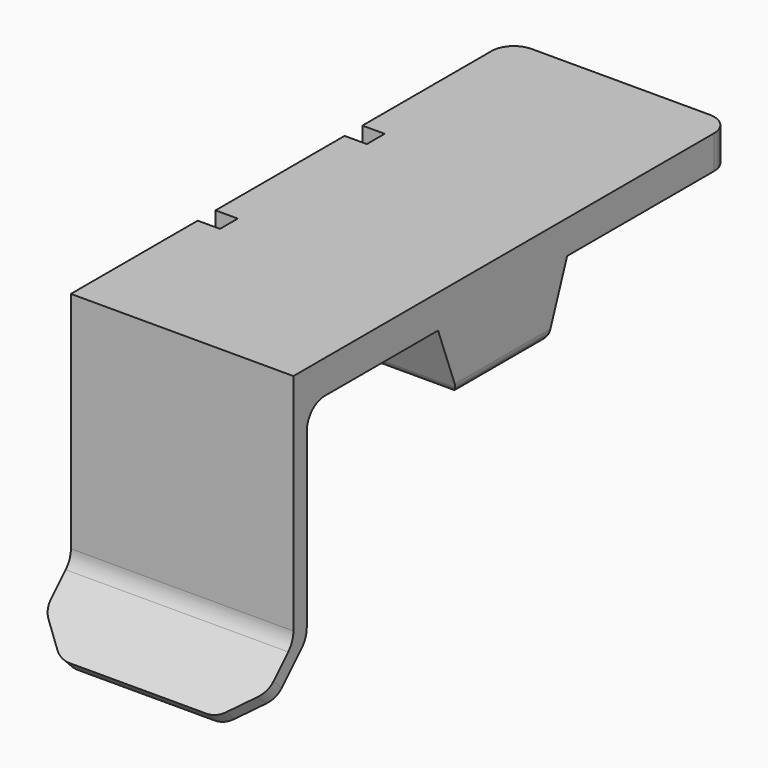
from build123d import *

# Parameters (mm, degrees)
F0_W         = 20
F0_H         = 47.7648153901
F1_DEPTH     = 3
F3_W         = 20
F3_H         = 23
F4_DEPTH     = 1.5
F5_T1_DEPTH  = 30.2867319519
F6_W         = 20
F6_H         = 2.1213203436
F7_DEPTH     = 7
F8_W         = 23.5785972327
F8_H         = 18.0557984859
F9_DEPTH     = 0.828
F10_SIZE     = 3
F11_R        = 2
F12_W        = 20
F12_H        = 16
F13_DEPTH    = 6
F14_T4_DEPTH = 61.5019292892
F14_T9_DEPTH = 61.5019292892
F15_R        = 2
F16_R        = 1
F17_W        = 2
F17_H        = 2
F18_DEPTH    = 3


# Not quite as in the source:
# - a fillet or chamfer that OpenCascade refuses, or shapes differently, is made with other operations: its cross-section is extruded or revolved along the edge and cut away or added


with BuildPart() as f1:
    # F0 (on Top) → F1 (new body)
    with BuildSketch(Plane.XY):
        Rectangle(F0_W, F0_H)
    extrude(amount=F1_DEPTH)

    # F3 (on offset) → F4 (join)
    with BuildSketch(Plane.XZ.offset(23.8824076951)):
        with Locations((0, -8.5)):
            Rectangle(F3_W, F3_H)
    extrude(amount=F4_DEPTH)

    # F5: chamfer of 2 on 1 edges, made by hand

    # F5_s2 → F5_t1 (cut)
    with BuildSketch(Plane.YZ.offset(-15.1433659759)):
        Polygon((-25.3824076951, -18), (-23.3824076951, -20), (-25.3824076951, -20), align=None)
    extrude(amount=F5_T1_DEPTH, mode=Mode.SUBTRACT)

    # F6 (on face) → F7 (join)
    with BuildSketch(Plane(origin=(0, -21.6912038475, -21.6912038475), x_dir=(1, 0, 0), z_dir=(0, -0.7071067812, -0.7071067812))):
        with Locations((0, 4.1594903709)):
            Rectangle(F6_W, F6_H)
    extrude(amount=F7_DEPTH)

    # F8 (on face) → F9 (cut)
    with BuildSketch(Plane(origin=(0, -2.1912038475, 2.1912038475), x_dir=(-1, 0, 0), z_dir=(0, 0.7071067812, -0.7071067812))):
        with Locations((-0.010414049, -33.0743109807)):
            Rectangle(F8_W, F8_H)
    extrude(amount=-F9_DEPTH, mode=Mode.SUBTRACT)

    # F10
    f10_edges = [f1.edges().sort_by_distance(p)[0] for p in [
        (-10, -29.874897, -23.407005),
        (10, -29.874897, -23.407005),
    ]]
    chamfer(f10_edges, length=F10_SIZE)

    # F11
    f11_edges = [f1.edges().sort_by_distance(p)[0] for p in [
        (0, -23.882408, 0),
        (0, -25.382408, -18),
        (0, -23.882408, -18.329031),
        (-10, -27.753577, -21.285685),
        (-7, -29.874897, -23.407005),
        (7, -29.874897, -23.407005),
        (10, -27.753577, -21.285685),
    ]]
    fillet(f11_edges, radius=F11_R)

    # F12 (on face) → F13 (join)
    with BuildSketch(Plane(origin=(0, 0, 0), x_dir=(1, 0, 0), z_dir=(0, 0, -1))):
        with Locations((0, 1.8824076951)):
            Rectangle(F12_W, F12_H)
    extrude(amount=F13_DEPTH)

    # F14: chamfer of 3 x 8 on 2 edges, made by hand


with BuildPart() as f14_tool2:
    # F14_s3 → F14_t4 (new body)
    with BuildSketch(Plane.YZ.offset(30.7509646446)):
        Polygon((-9.8824076951, 2), (-6.8824076951, -6), (-9.8824076951, -6), align=None)
    extrude(amount=-F14_T4_DEPTH)

    split(bisect_by=Plane.XY, keep=Keep.BOTTOM)


with BuildPart() as f1_1:
    add(f1.part)

    # F14_t1: cut F14_tool2
    add(f14_tool2.part, mode=Mode.SUBTRACT)


with BuildPart() as f14_tool7:
    # F14_s8 → F14_t9 (new body)
    with BuildSketch(Plane.YZ.offset(-30.7509646446)):
        Polygon((6.1175923049, 2), (3.1175923049, -6), (6.1175923049, -6), align=None)
    extrude(amount=F14_T9_DEPTH)

    split(bisect_by=Plane.XY, keep=Keep.BOTTOM)


with BuildPart() as f1_2:
    add(f1_1.part)

    # F14_t6: cut F14_tool7
    add(f14_tool7.part, mode=Mode.SUBTRACT)

    # F15
    f15_edges = [f1_2.edges().sort_by_distance(p)[0] for p in [
        (-10, 23.882408, 1.5),
        (10, 23.882408, 1.5),
    ]]
    fillet(f15_edges, radius=F15_R)

    # F16
    f16_edges = [f1_2.edges().sort_by_distance(p)[0] for p in [
        (-10, -1.882408, -6),
        (0, -6.882408, -6),
        (10, -1.882408, -6),
        (0, 3.117592, -6),
    ]]
    fillet(f16_edges, radius=F16_R)

    # F17 (on face) → F18 (cut, through all)
    with BuildSketch(Plane(origin=(0, 0, 0), x_dir=(1, 0, 0), z_dir=(0, 0, -1))):
        with Locations((-9, -6.3675923049)):
            Rectangle(F17_W, F17_H)
        with Locations((-9, 10.1324076951)):
            Rectangle(F17_W, F17_H)
    extrude(amount=-F18_DEPTH, mode=Mode.SUBTRACT)


solid = f1_2.part
